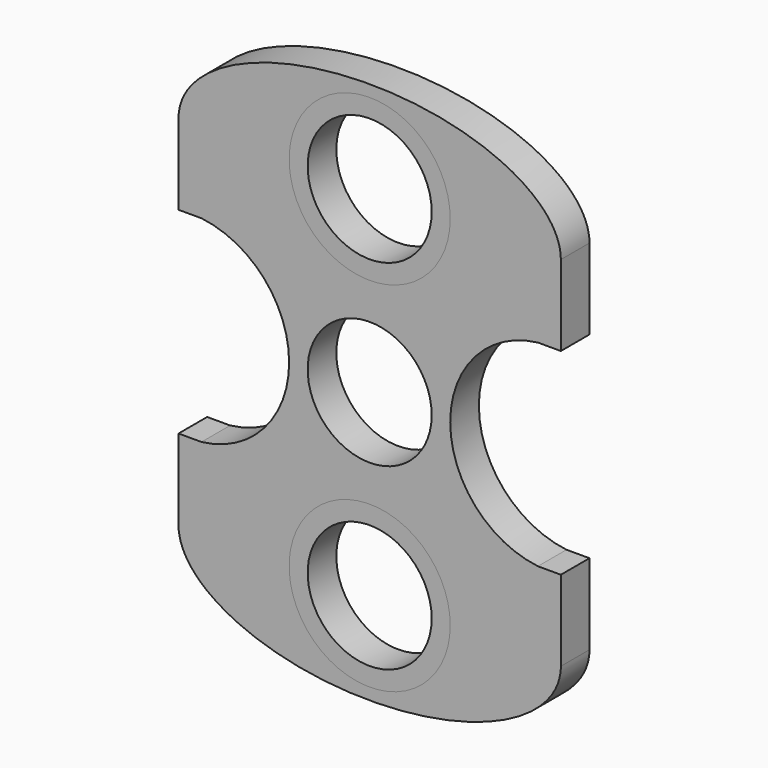
from build123d import *

# Parameters (mm, degrees)
F1_R     = 10.9982
F1_R_2   = 14.2875
F2_DEPTH = 6.35
F0_R     = 14.2875
F0_R_2   = 10.9982


with BuildPart() as f2:
    # F1 (on Front) → F2 (new body)
    with BuildSketch(Plane.XZ):
        with BuildLine():
            Line((-33.9049473405, 17.4625), (-29.8317704118, 17.4625))
            ThreePointArc((-29.8317704118, 17.4625), (-31.8683588761, 17.5808588761), (-33.9049473405, 17.4625))
        make_face()
        with BuildLine():
            ThreePointArc((-33.9049473405, -17.4625), (-31.8683588761, -17.5808588761), (-29.8317704118, -17.4625))
            Line((-29.8317704118, -17.4625), (-33.9049473405, -17.4625))
        make_face()
        with BuildLine():
            ThreePointArc((33.9049473405, 17.4625), (31.8683588761, 17.5808588761), (29.8317704118, 17.4625))
            Line((29.8317704118, 17.4625), (33.9049473405, 17.4625))
        make_face()
        with BuildLine():
            Line((33.9049473405, -17.4625), (29.8317704118, -17.4625))
            ThreePointArc((29.8317704118, -17.4625), (31.8683588761, -17.5808588761), (33.9049473405, -17.4625))
        make_face()
        with BuildLine():
            ThreePointArc((-14.2875, 1.47e-08), (-7.3e-09, -14.2875), (14.2875, 0))
            ThreePointArc((14.2875, 0), (7.3e-09, 14.2875), (-14.2875, 1.47e-08))
        make_face()
        Circle(F1_R, mode=Mode.SUBTRACT)
        with BuildLine():
            ThreePointArc((29.8317704118, -17.4625), (18.7364973706, -11.689346099), (14.2875, 0))
            ThreePointArc((14.2875, 0), (-7.3e-09, -14.2875), (-14.2875, 1.47e-08))
            ThreePointArc((-14.2875, 1.47e-08), (-18.7364973657, -11.6893460935), (-29.8317704118, -17.4625))
            ThreePointArc((-29.8317704118, -17.4625), (-31.8683588761, -17.5808588761), (-33.9049473405, -17.4625))
            Line((-33.9049473405, -17.4625), (-33.9049473405, -31.75))
            add(Edge.make_bspline(
                [(-33.9049473405, -31.75), (-33.9049473405, -48.1233965864), (0, -48.1233965864), (33.9049473405, -48.1233965864), (33.9049473405, -31.75)],
                knots=[3.1415926536, 3.1415926536, 3.1415926536, 4.7123889804, 4.7123889804, 6.2831853072, 6.2831853072, 6.2831853072], degree=2, weights=[1, 0.7071067812, 1, 0.7071067812, 1]))
            Line((33.9049473405, -31.75), (33.9049473405, -17.4625))
            ThreePointArc((33.9049473405, -17.4625), (31.8683588761, -17.5808588761), (29.8317704118, -17.4625))
        make_face()
        with Locations((0, -31.75)):
            Circle(F1_R_2, mode=Mode.SUBTRACT)
        with BuildLine():
            ThreePointArc((-14.2875, 1.47e-08), (7.3e-09, 14.2875), (14.2875, 0))
            ThreePointArc((14.2875, 0), (18.7364973706, 11.689346099), (29.8317704118, 17.4625))
            ThreePointArc((29.8317704118, 17.4625), (31.8683588761, 17.5808588761), (33.9049473405, 17.4625))
            Line((33.9049473405, 17.4625), (33.9049473405, 31.75))
            add(Edge.make_bspline(
                [(33.9049473405, 31.75), (33.9049473405, 48.1233965864), (0, 48.1233965864), (-33.9049473405, 48.1233965864), (-33.9049473405, 31.75)],
                knots=[3.1415926536, 3.1415926536, 3.1415926536, 4.7123889804, 4.7123889804, 6.2831853072, 6.2831853072, 6.2831853072], degree=2, weights=[1, 0.7071067812, 1, 0.7071067812, 1]))
            Line((-33.9049473405, 31.75), (-33.9049473405, 17.4625))
            ThreePointArc((-33.9049473405, 17.4625), (-31.8683588761, 17.5808588761), (-29.8317704118, 17.4625))
            ThreePointArc((-29.8317704118, 17.4625), (-18.7364973754, 11.6893461044), (-14.2875, 1.47e-08))
        make_face()
        with BuildLine():
            ThreePointArc((-14.2875, 31.75), (0, 46.0375), (14.2875, 31.75))
            ThreePointArc((14.2875, 31.75), (0, 17.4625), (-14.2875, 31.75))
        make_face(mode=Mode.SUBTRACT)
    extrude(amount=F2_DEPTH)


with BuildPart() as f2b:
    # F0 (on Front) → F2, piece 2 (new body)
    with BuildSketch(Plane.XZ):
        with Locations((0, 31.75)):
            Circle(F0_R)
        with Locations((0, 31.75)):
            Circle(F0_R_2, mode=Mode.SUBTRACT)
    extrude(amount=F2_DEPTH)


with BuildPart() as f2c:
    # F0 (on Front) → F2, piece 3 (new body)
    with BuildSketch(Plane.XZ):
        with Locations((0, -31.75)):
            Circle(F0_R)
        with Locations((0, -31.75)):
            Circle(F0_R_2, mode=Mode.SUBTRACT)
    extrude(amount=F2_DEPTH)


solid = Compound([f2.part, f2b.part, f2c.part])
